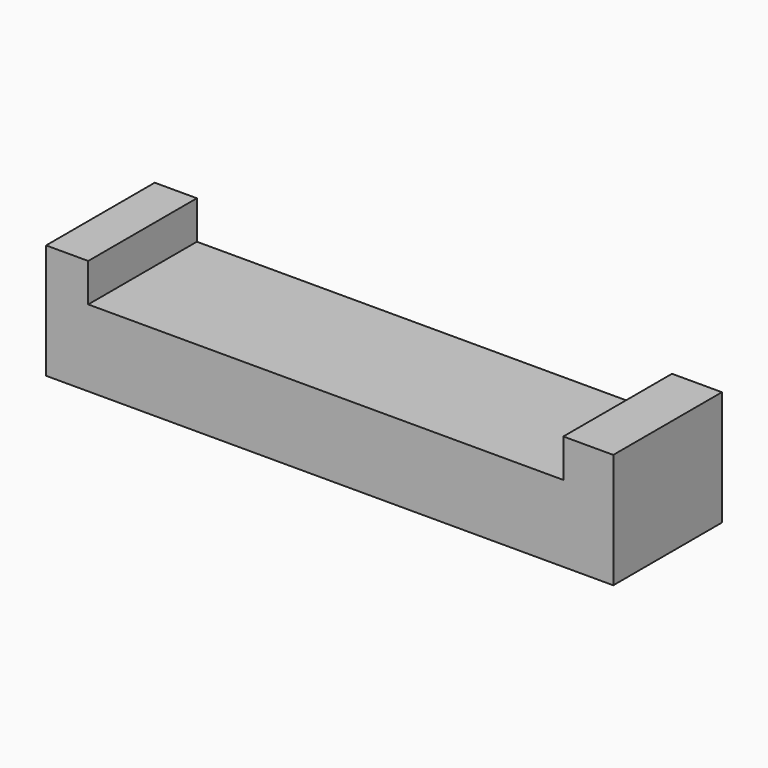
from build123d import *

# Parameters (mm, degrees)
F0_W         = 74.1065517068
F0_H         = 17.7458450198
F1_DEPTH     = 10
F2_W         = 5.5062570609
F2_H         = 17.7458450198
F2_W_2       = 6.5232515335
F3_DEPTH     = 5
F4_TEXT_SIZE = 3.8798154694
F5_DEPTH     = 5


# Not quite as in the source:
# - Text() gives the source's letters only with a copy of the font that has no kerning and outlines rounded to 1/6400 em; it was checked with that copy


with BuildPart() as f1:
    # F0 (on Top) → F1 (new body)
    with BuildSketch(Plane.XY):
        with Locations((37.0532758534, 8.8729225099)):
            Rectangle(F0_W, F0_H)
    extrude(amount=F1_DEPTH)

    # F2 (on face) → F3 (join)
    with BuildSketch(Plane.XY.offset(10)):
        with Locations((2.7531285305, 8.8729225099)):
            Rectangle(F2_W, F2_H)
        with Locations((70.84492594, 8.8729225099)):
            Rectangle(F2_W_2, F2_H)
    extrude(amount=F3_DEPTH)

    # F4 (on face) → F5 (cut)
    with BuildSketch(Plane(origin=(0, 0, 0), x_dir=(1, 0, 0), z_dir=(0, 0, -1))):
        with Locations((16.7618445121, -8.4461420774)):
            Text('Send Purchase Request', F4_TEXT_SIZE, font='Open Sans', text_align=(TextAlign.LEFT, TextAlign.BOTTOM))
    extrude(amount=-F5_DEPTH, mode=Mode.SUBTRACT)


solid = f1.part
